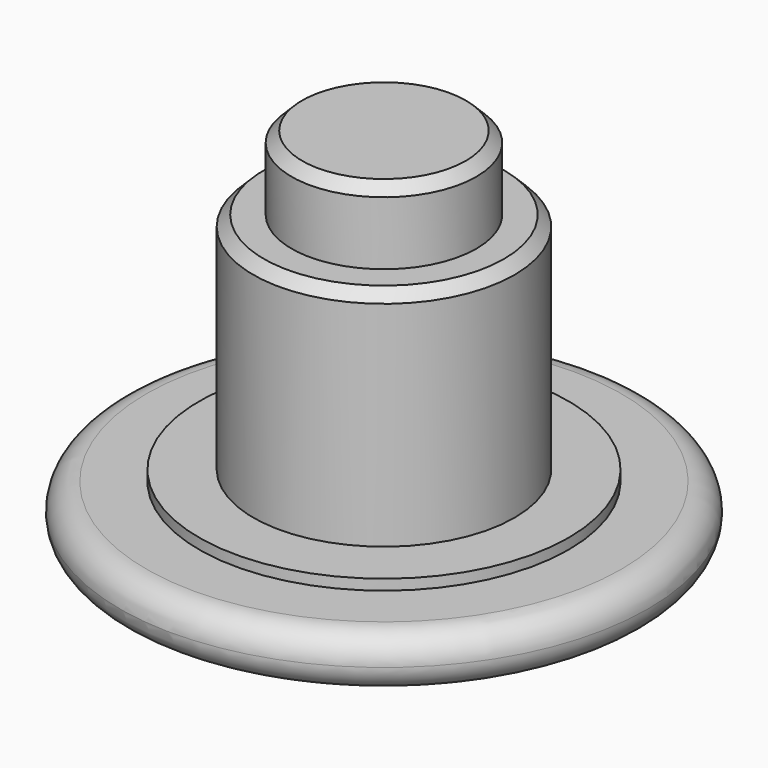
from build123d import *

# Parameters (mm, degrees)
F0_R     = 4.95
F1_DEPTH = 8.5
F2_R     = 7
F3_DEPTH = 0.4
F4_R     = 10
F5_DEPTH = 2
F6_R     = 0.99999
F7_R     = 3.5
F8_DEPTH = 2.8
F9_SIZE  = 0.4


# Not quite as in the source:
# - a fillet or chamfer is up to 0.001 mm smaller than in the source, because OpenCascade refuses the exact size


with BuildPart() as f1:
    # F0 (on Top) → F1 (new body)
    with BuildSketch(Plane.XY):
        Circle(F0_R)
    extrude(amount=F1_DEPTH)

    # F2 (on Top) → F3 (join)
    with BuildSketch(Plane.XY):
        Circle(F2_R)
    extrude(amount=-F3_DEPTH)

    # F4 (on face) → F5 (join)
    with BuildSketch(Plane(origin=(0, 0, -0.4), x_dir=(1, 0, 0), z_dir=(0, 0, -1))):
        Circle(F4_R)
    extrude(amount=F5_DEPTH)

    # F6 (radius 1 in the source; OpenCascade refuses exactly that, so slightly less here)
    f6_edges = [f1.edges().sort_by_distance(p)[0] for p in [
        (-10, 0, -2.4),
        (-10, 0, -0.4),
    ]]
    fillet(f6_edges, radius=F6_R)

    # F7 (on face) → F8 (join)
    with BuildSketch(Plane.XY.offset(8.5)):
        Circle(F7_R)
    extrude(amount=F8_DEPTH)

    # F9
    f9_edges = [f1.edges().sort_by_distance(p)[0] for p in [
        (-3.5, 0, 11.3),
        (-4.95, 0, 8.5),
    ]]
    chamfer(f9_edges, length=F9_SIZE)


solid = f1.part
